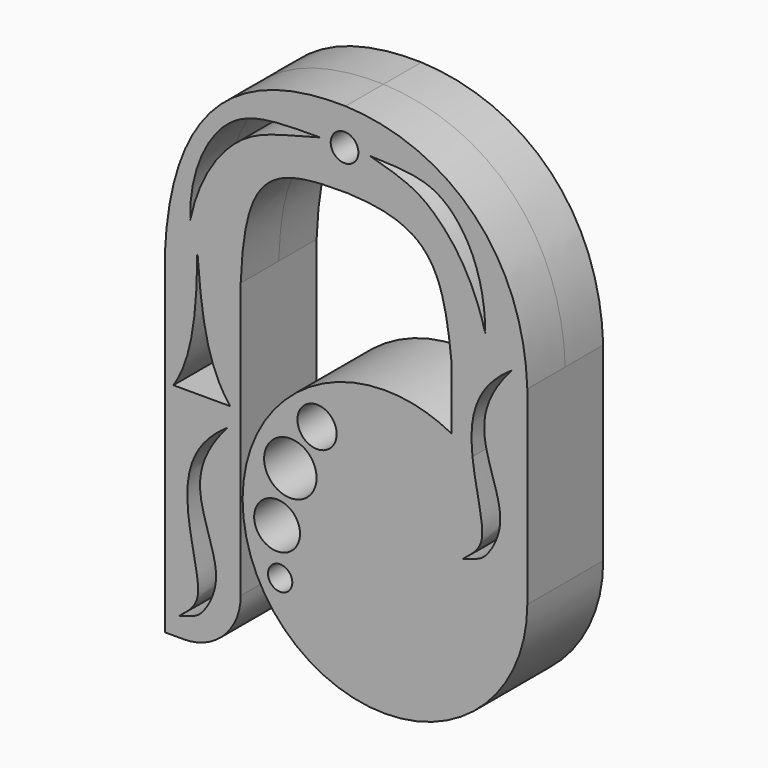
from build123d import *

# Parameters (mm, degrees)
F1_DEPTH = 6.35
F2_R     = 7.62
F3_R     = 1.851317794
F3_R_2   = 2.623048948
F3_R_3   = 3.5099243314
F3_R_4   = 3.0648100187
F3_R_5   = 1.624839295
F4_DEPTH = 12.7


# Not quite as in the source:
# - a feature names something its author has since deleted; it is built from what else it names


with BuildPart() as f1:
    # F0 (on Front) → F1 (new body, symmetric)
    with BuildSketch(Plane.XZ):
        with BuildLine():
            Line((-47.4034676004, -12.1683157229), (-47.4034676004, -56.6183157229))
            Line((-47.4034676004, -56.6183157229), (-37.2434676004, -56.6183157229))
            Line((-37.2434676004, -56.6183157229), (-37.2434676004, -12.1683157229))
            add(Edge.make_bspline(
                [(-37.2434676004, -12.1683157229), (-36.7095838945, 1.4708520701), (-33.3203151822, 3.1873958426), (-22.9693437804, 3.0716842771)],
                knots=[0, 0, 0, 0, 20.8808096306, 20.8808096306, 20.8808096306, 20.8808096306], degree=3))
            add(Edge.make_bspline(
                [(-22.9693437804, 3.0716842771), (-11.9594718681, 2.6847659899), (-10.1360433424, -1.6166193699), (-9.0494676004, -12.1683158262)],
                knots=[0, 0, 0, 0, 20.6402654057, 20.6402654057, 20.6402654057, 20.6402654057], degree=3))
            Line((-9.0494676004, -12.1683158262), (-9.0494676004, -20.7198617879))
            ThreePointArc((-9.0494676004, -20.7198617879), (-7.6000300221, -21.5683616428), (-6.2309603269, -22.5412282663))
            add(Edge.make_bspline(
                [(-6.2309603269, -22.5412282663), (-6.2723652172, -22.1636683346), (-6.6533718861, -17.8378431816), (-5.6407446666, -13.777271871), (-0.9912915077, -10.6814840494)],
                knots=[0.5669230938, 0.5669230938, 0.5669230938, 0.5669230938, 0.6047158912, 1, 1, 1, 1], degree=3))
            add(Edge.make_bspline(
                [(-2.9873109532, -25.7642693151), (-3.3866343808, -24.3019783121), (-5.124946874, -19.6083809219), (-4.8990877844, -15.1703206189), (-0.9912915077, -10.6814840494)],
                knots=[0.5181753665, 0.5181753665, 0.5181753665, 0.5181753665, 0.6734400418, 1, 1, 1, 1], degree=3))
            ThreePointArc((-2.9873109532, -25.7642693151), (0.0569359866, -31.3207595659), (1.1105323996, -37.5683157229))
            Line((1.1105323996, -37.5683157229), (1.1105323996, -12.1683157229))
            add(Edge.make_bspline(
                [(1.1105323996, -12.1683157229), (0.5705629619, 4.0617453953), (-10.3604181223, 12.7446337565), (-23.2162306761, 13.2316842771)],
                knots=[0, 0, 0, 0, 35.1703198982, 35.1703198982, 35.1703198982, 35.1703198982], degree=3))
            add(Edge.make_bspline(
                [(-47.4034676004, -12.1683157229), (-46.5849920508, 7.3050484799), (-36.5418703402, 13.5184679613), (-23.2162306761, 13.2316842771)],
                knots=[0, 0, 0, 0, 35.0739565779, 35.0739565779, 35.0739565779, 35.0739565779], degree=3))
        make_face()
        with BuildLine():
            add(Edge.make_bspline(
                [(-45.5194190145, -54.1016533971), (-43.4073472429, -53.4859708194), (-42.3767122517, -53.0275311605), (-39.4416086551, -47.8736285865), (-43.2098006647, -39.8360561852), (-42.9273473132, -34.2859363798), (-39.0195510365, -29.7970998103)],
                knots=[0, 0, 0, 0, 0.1860018813, 0.3974429686, 0.6734400418, 1, 1, 1, 1], degree=3))
            add(Edge.make_bspline(
                [(-45.5194190145, -54.1016533971), (-43.4073472429, -52.4910938487), (-42.1962339672, -50.3443092376), (-45.4188846713, -39.9097980212), (-43.6690041954, -32.8928876319), (-39.0195510365, -29.7970998103)],
                knots=[0, 0, 0, 0, 0.2516171716, 0.6047158912, 1, 1, 1, 1], degree=3))
        make_face(mode=Mode.SUBTRACT)
        with BuildLine():
            add(Edge.make_bspline(
                [(-43.0450886488, -10.2955098264), (-43.0850870907, -18.8955254853), (-44.0450869501, -23.7755347043), (-46.2450906634, -27.1355397999)],
                knots=[0, 0, 0, 0, 17.1413716605, 17.1413716605, 17.1413716605, 17.1413716605], degree=3))
            add(Edge.make_bspline(
                [(-43.0450886488, -10.2955098264), (-42.4450859427, -18.8155258074), (-41.4850823581, -23.4555341303), (-38.685079664, -27.1355397999)],
                knots=[0, 0, 0, 0, 17.395294992, 17.395294992, 17.395294992, 17.395294992], degree=3))
            Line((-38.685079664, -27.1355397999), (-46.2450906634, -27.1355397999))
        make_face(mode=Mode.SUBTRACT)
        with BuildLine():
            add(Edge.make_bspline(
                [(-43.9962111413, -6.9482689141), (-42.8800281093, -1.4789610887), (-37.594435646, 6.055033296), (-32.2294885174, 6.9111710616), (-26.6296397895, 8.4384027869)],
                knots=[0, 0, 0, 0, 0.5184862256, 1, 1, 1, 1], degree=3))
            add(Edge.make_bspline(
                [(-43.9962111413, -6.9482689141), (-44.1630539416, -1.2757268376), (-39.7049183871, 8.2866771022), (-32.6861925423, 8.4215123206), (-26.6296397895, 8.4384027869)],
                knots=[0, 0, 0, 0, 0.513875061, 1, 1, 1, 1], degree=3))
        make_face(mode=Mode.SUBTRACT)
        with BuildLine():
            add(Edge.make_bspline(
                [(-19.9744962156, 8.4384027869), (-15.0681919771, 7.110938792), (-11.4060719241, 5.2750660976), (-6.2541036922, -1.0550173553), (-4.5138360001, -7.4359978316)],
                knots=[0, 0, 0, 0, 0.4513191083, 1, 1, 1, 1], degree=3))
            add(Edge.make_bspline(
                [(-19.9744962156, 8.4384027869), (-14.4520029301, 8.3067857058), (-9.1414830202, 7.6395398298), (-4.5325819981, -0.7140918586), (-4.5138360001, -7.4359978316)],
                knots=[0, 0, 0, 0, 0.4604709536, 1, 1, 1, 1], degree=3))
        make_face(mode=Mode.SUBTRACT)
        with BuildLine():
            ThreePointArc((-17.9394676004, -18.5183157229), (-31.409851782, -24.0979315413), (-36.9894676004, -37.5683157229))
            Line((-36.9894676004, -37.5683157229), (-17.9394676004, -37.5683157229))
            Line((-17.9394676004, -37.5683157229), (-17.9394676004, -18.5183157229))
        make_face()
        with BuildLine():
            ThreePointArc((-17.9394676004, -56.6183157229), (-4.4690834188, -51.0386999045), (1.1105323996, -37.5683157229))
            ThreePointArc((1.1105323996, -37.5683157229), (0.0569359866, -31.3207595659), (-2.9873109532, -25.7642693151))
            add(Edge.make_bspline(
                [(-7.4911594857, -34.9860376362), (-5.3790877141, -34.3703550585), (-4.3484527229, -33.9119153996), (-2.0900506569, -29.9462685874), (-2.6768006917, -26.9013334848), (-2.9873109532, -25.7642693151)],
                knots=[0, 0, 0, 0, 0.1860018813, 0.3974429686, 0.5181753665, 0.5181753665, 0.5181753665, 0.5181753665], degree=3))
            add(Edge.make_bspline(
                [(-7.4911594857, -34.9860376362), (-5.3790877141, -33.3754780878), (-4.243665121, -31.362860607), (-5.8855186547, -25.6912169104), (-6.2309603269, -22.5412282663)],
                knots=[0, 0, 0, 0, 0.2516171716, 0.5669230938, 0.5669230938, 0.5669230938, 0.5669230938], degree=3))
            ThreePointArc((-6.2309603269, -22.5412282663), (-7.6000300221, -21.5683616428), (-9.0494676004, -20.7198617879))
            ThreePointArc((-9.0494676004, -20.7198617879), (-13.3601962316, -19.0768913935), (-17.9394676004, -18.5183157229))
            Line((-17.9394676004, -18.5183157229), (-17.9394676004, -37.5683157229))
            Line((-17.9394676004, -37.5683157229), (-17.9394676004, -56.6183157229))
        make_face()
        with BuildLine():
            ThreePointArc((-36.9894676004, -37.5683157229), (-31.409851782, -51.0386999045), (-17.9394676004, -56.6183157229))
            Line((-17.9394676004, -56.6183157229), (-17.9394676004, -37.5683157229))
            Line((-17.9394676004, -37.5683157229), (-36.9894676004, -37.5683157229))
        make_face()
    extrude(amount=F1_DEPTH, both=True)

    # F2
    f2_edges = [f1.edges().sort_by_distance(p)[0] for p in [
        (-37.243468, 0, -56.618316),
    ]]
    fillet(f2_edges, radius=F2_R)

    # F3 (on Front) → F4 (cut, symmetric)
    with BuildSketch(Plane.XZ):
        with Locations((-23.3467891812, 8.3186188713)):
            Circle(F3_R)
        with Locations((-27.0257256925, -25.7905125618)):
            Circle(F3_R_2)
        with Locations((-30.5994562805, -31.8327024579)):
            Circle(F3_R_3)
        with Locations((-32.374959439, -39.1334928572)):
            Circle(F3_R_4)
        with Locations((-31.9626331329, -45.2065691352)):
            Circle(F3_R_5)
    extrude(amount=F4_DEPTH, both=True, mode=Mode.SUBTRACT)


solid = f1.part
